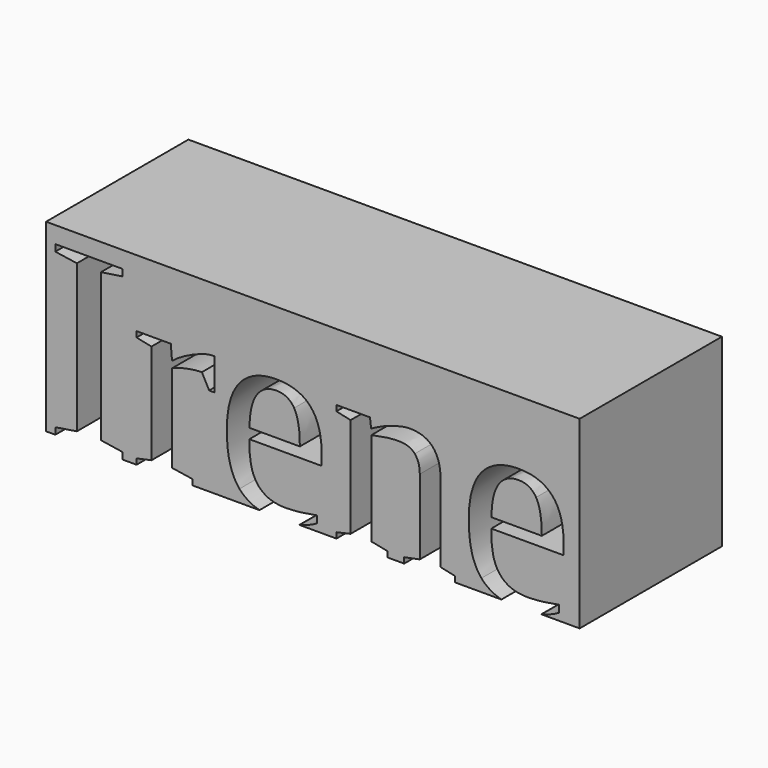
from build123d import *

# Parameters (mm, degrees)
F1_DEPTH = 25.4


with BuildPart() as f1:
    # F0 (on Front) → F1 (new body)
    with BuildSketch(Plane.XZ):
        with BuildLine():
            Line((37.3974812319, 27.1067991487), (-38.8025187681, 27.1067991487))
            Line((-38.8025187681, 27.1067991487), (-38.8025187681, 0.7496755936))
            Line((-38.8025187681, 0.7496755936), (-37.4812306732, 0.7496755936))
            Line((-37.4812306732, 0.7496755936), (-37.4812306732, 1.6991726661))
            Line((-37.4812306732, 1.6991726661), (-34.4039449803, 2.1796410643))
            Line((-34.4039449803, 2.1796410643), (-34.4039449803, 23.3088108586))
            Line((-34.4039449803, 23.3088108586), (-37.4812306732, 23.7721196711))
            Line((-37.4812306732, 23.7721196711), (-37.4812306732, 24.7216167436))
            Line((-37.4812306732, 24.7216167436), (-27.9004620198, 24.7216167436))
            Line((-27.9004620198, 24.7216167436), (-27.9004620198, 23.7721196711))
            Line((-27.9004620198, 23.7721196711), (-30.9720278508, 23.3088108586))
            Line((-30.9720278508, 23.3088108586), (-30.9720278508, 2.1796410643))
            Line((-30.9720278508, 2.1796410643), (-27.9004620198, 1.6991726661))
            Line((-27.9004620198, 1.6991726661), (-27.9004620198, 0.7496755936))
            Line((-27.9004620198, 0.7496755936), (-25.8813507753, 0.7496755936))
            Line((-25.8813507753, 0.7496755936), (-25.8813507753, 1.5561761191))
            Line((-25.8813507753, 1.5561761191), (-23.7535621549, 2.0023253459))
            Line((-23.7535621549, 2.0023253459), (-23.7535621549, 16.3019800524))
            Line((-23.7535621549, 16.3019800524), (-25.8813507753, 16.7481292793))
            Line((-25.8813507753, 16.7481292793), (-25.8813507753, 17.5546298047))
            Line((-25.8813507753, 17.5546298047), (-20.9851490038, 17.5546298047))
            Line((-20.9851490038, 17.5546298047), (-20.8192730092, 15.4611603557))
            add(Edge.make_bspline(
                [(-20.8192730092, 15.4611603557), (-19.7496588371, 16.3534588094), (-17.9164431038, 17.1771189205)],
                knots=[0, 0, 0, 1, 1, 1], degree=2))
            add(Edge.make_bspline(
                [(-17.9164431038, 17.1771189205), (-16.0832273704, 18.0007790316), (-15.0136131983, 18.0007790316)],
                knots=[0, 0, 0, 1, 1, 1], degree=2))
            Line((-15.0136131983, 18.0007790316), (-14.7447796899, 18.0007790316))
            Line((-14.7447796899, 18.0007790316), (-14.7447796899, 13.4592086968))
            Line((-14.7447796899, 13.4592086968), (-15.5112411821, 13.4592086968))
            Line((-15.5112411821, 13.4592086968), (-16.5522560448, 15.4268411844))
            add(Edge.make_bspline(
                [(-16.5522560448, 15.4268411844), (-17.4445544984, 15.4268411844), (-18.6686049413, 15.1837470544)],
                knots=[0, 0, 0, 1, 1, 1], degree=2))
            add(Edge.make_bspline(
                [(-18.6686049413, 15.1837470544), (-19.8926553842, 14.9406529244), (-20.7849538379, 14.5517023164)],
                knots=[0, 0, 0, 1, 1, 1], degree=2))
            Line((-20.7849538379, 14.5517023164), (-20.7849538379, 2.0023253459))
            Line((-20.7849538379, 2.0023253459), (-17.9078633109, 1.5561761191))
            Line((-17.9078633109, 1.5561761191), (-17.9078633109, 0.7496755936))
            Line((-17.9078633109, 0.7496755936), (-8.3285276719, 0.7496755936))
            add(Edge.make_bspline(
                [(-8.3285276719, 0.7496755936), (-10.11731664, 1.2614297437), (-11.181305737, 2.4999533297)],
                knots=[0.4131969353, 0.4131969353, 0.4131969353, 1, 1, 1], degree=2))
            add(Edge.make_bspline(
                [(-11.181305737, 2.4999533297), (-12.9945019538, 4.6105823644), (-12.9945019538, 9.2779896606)],
                knots=[0, 0, 0, 1, 1, 1], degree=2))
            add(Edge.make_bspline(
                [(-12.9945019538, 9.2779896606), (-12.9945019538, 13.6708435864), (-11.1527064276, 15.835811309)],
                knots=[0, 0, 0, 1, 1, 1], degree=2))
            add(Edge.make_bspline(
                [(-11.1527064276, 15.835811309), (-9.3109109014, 18.0007790316), (-5.8961533575, 18.0007790316)],
                knots=[0, 0, 0, 1, 1, 1], degree=2))
            add(Edge.make_bspline(
                [(-5.8961533575, 18.0007790316), (0.5558508461, 18.0007790316), (0.5558508461, 10.6679160981)],
                knots=[0, 0, 0, 1, 1, 1], degree=2))
            Line((0.5558508461, 10.6679160981), (0.5558508461, 9.2036314561))
            Line((0.5558508461, 9.2036314561), (-9.7742197139, 9.2036314561))
            Line((-9.7742197139, 9.2036314561), (-9.7742197139, 8.8833191907))
            add(Edge.make_bspline(
                [(-9.7742197139, 8.8833191907), (-9.7742197139, 6.4180587193), (-9.230832835, 5.0510117294)],
                knots=[0, 0, 0, 1, 1, 1], degree=2))
            add(Edge.make_bspline(
                [(-9.230832835, 5.0510117294), (-8.6874459562, 3.6839647394), (-7.5520533725, 2.9689820041)],
                knots=[0, 0, 0, 1, 1, 1], degree=2))
            add(Edge.make_bspline(
                [(-7.5520533725, 2.9689820041), (-6.4166607888, 2.2539992688), (-4.5748652626, 2.2539992688)],
                knots=[0, 0, 0, 1, 1, 1], degree=2))
            add(Edge.make_bspline(
                [(-4.5748652626, 2.2539992688), (-3.6082086044, 2.2539992688), (-2.2869205095, 2.4141554015)],
                knots=[0, 0, 0, 1, 1, 1], degree=2))
            add(Edge.make_bspline(
                [(-2.2869205095, 2.4141554015), (-0.9656324147, 2.5743115342), (-0.1076531323, 2.7687868382)],
                knots=[0, 0, 0, 1, 1, 1], degree=2))
            Line((-0.1076531323, 2.7687868382), (-0.1076531323, 1.7678110087))
            add(Edge.make_bspline(
                [(-0.1076531323, 1.7678110087), (-0.9656324147, 1.2129844061), (-2.4384968494, 0.8011543506)],
                knots=[0, 0, 0, 1, 1, 1], degree=2))
            add(Edge.make_bspline(
                [(-2.4384968494, 0.8011543506), (-2.5336227612, 0.7745560374), (-2.6290230549, 0.7496755936)],
                knots=[0, 0, 0, 0.0645856533, 0.0645856533, 0.0645856533], degree=2))
            Line((-2.6290230549, 0.7496755936), (2.6664798808, 0.7496755936))
            Line((2.6664798808, 0.7496755936), (2.6664798808, 1.5561761191))
            Line((2.6664798808, 1.5561761191), (4.6855911253, 2.0023253459))
            Line((4.6855911253, 2.0023253459), (4.6855911253, 16.3019800524))
            Line((4.6855911253, 16.3019800524), (2.6664798808, 16.7481292793))
            Line((2.6664798808, 16.7481292793), (2.6664798808, 17.5546298047))
            Line((2.6664798808, 17.5546298047), (7.4540042765, 17.5546298047))
            Line((7.4540042765, 17.5546298047), (7.6198802711, 16.1933026767))
            add(Edge.make_bspline(
                [(7.6198802711, 16.1933026767), (8.9926471229, 16.9826436165), (10.548449555, 17.491711324)],
                knots=[0, 0, 0, 1, 1, 1], degree=2))
            add(Edge.make_bspline(
                [(10.548449555, 17.491711324), (12.1042519871, 18.0007790316), (13.1395469878, 18.0007790316)],
                knots=[0, 0, 0, 1, 1, 1], degree=2))
            add(Edge.make_bspline(
                [(13.1395469878, 18.0007790316), (15.3188143651, 18.0007790316), (16.4284675703, 16.7309696936)],
                knots=[0, 0, 0, 1, 1, 1], degree=2))
            add(Edge.make_bspline(
                [(16.4284675703, 16.7309696936), (17.5381207755, 15.4611603557), (17.5381207755, 13.0473786412)],
                knots=[0, 0, 0, 1, 1, 1], degree=2))
            Line((17.5381207755, 13.0473786412), (17.5381207755, 2.0023253459))
            Line((17.5381207755, 2.0023253459), (19.5743916057, 1.5561761191))
            Line((19.5743916057, 1.5561761191), (19.5743916057, 0.7496755936))
            Line((19.5743916057, 0.7496755936), (26.2251579609, 0.7496755936))
            add(Edge.make_bspline(
                [(26.2251579609, 0.7496755936), (24.4363689928, 1.2614297437), (23.3723798958, 2.4999533297)],
                knots=[0.4131969353, 0.4131969353, 0.4131969353, 1, 1, 1], degree=2))
            add(Edge.make_bspline(
                [(23.3723798958, 2.4999533297), (21.559183679, 4.6105823644), (21.559183679, 9.2779896606)],
                knots=[0, 0, 0, 1, 1, 1], degree=2))
            add(Edge.make_bspline(
                [(21.559183679, 9.2779896606), (21.559183679, 13.6708435864), (23.4009792052, 15.835811309)],
                knots=[0, 0, 0, 1, 1, 1], degree=2))
            add(Edge.make_bspline(
                [(23.4009792052, 15.835811309), (25.2427747314, 18.0007790316), (28.6575322753, 18.0007790316)],
                knots=[0, 0, 0, 1, 1, 1], degree=2))
            add(Edge.make_bspline(
                [(28.6575322753, 18.0007790316), (35.1095364789, 18.0007790316), (35.1095364789, 10.6679160981)],
                knots=[0, 0, 0, 1, 1, 1], degree=2))
            Line((35.1095364789, 10.6679160981), (35.1095364789, 9.2036314561))
            Line((35.1095364789, 9.2036314561), (24.7794659189, 9.2036314561))
            Line((24.7794659189, 9.2036314561), (24.7794659189, 8.8833191907))
            add(Edge.make_bspline(
                [(24.7794659189, 8.8833191907), (24.7794659189, 6.4180587193), (25.3228527978, 5.0510117294)],
                knots=[0, 0, 0, 1, 1, 1], degree=2))
            add(Edge.make_bspline(
                [(25.3228527978, 5.0510117294), (25.8662396766, 3.6839647394), (27.0016322603, 2.9689820041)],
                knots=[0, 0, 0, 1, 1, 1], degree=2))
            add(Edge.make_bspline(
                [(27.0016322603, 2.9689820041), (28.137024844, 2.2539992688), (29.9788203702, 2.2539992688)],
                knots=[0, 0, 0, 1, 1, 1], degree=2))
            add(Edge.make_bspline(
                [(29.9788203702, 2.2539992688), (30.9454770284, 2.2539992688), (32.2667651232, 2.4141554015)],
                knots=[0, 0, 0, 1, 1, 1], degree=2))
            add(Edge.make_bspline(
                [(32.2667651232, 2.4141554015), (33.5880532181, 2.5743115342), (34.4460325005, 2.7687868382)],
                knots=[0, 0, 0, 1, 1, 1], degree=2))
            Line((34.4460325005, 2.7687868382), (34.4460325005, 1.7678110087))
            add(Edge.make_bspline(
                [(34.4460325005, 1.7678110087), (33.5880532181, 1.2129844061), (32.1151887834, 0.8011543506)],
                knots=[0, 0, 0, 1, 1, 1], degree=2))
            add(Edge.make_bspline(
                [(32.1151887834, 0.8011543506), (32.0200628716, 0.7745560374), (31.9246625779, 0.7496755936)],
                knots=[0, 0, 0, 0.0645856533, 0.0645856533, 0.0645856533], degree=2))
            Line((31.9246625779, 0.7496755936), (37.3974812319, 0.7496755936))
            Line((37.3974812319, 0.7496755936), (37.3974812319, 27.1067991487))
        make_face()
    extrude(amount=F1_DEPTH)


with BuildPart() as f1b:
    # F0 (on Front) → F1, piece 2 (new body)
    with BuildSketch(Plane.XZ):
        with BuildLine():
            Line((9.9249846098, 0.7496755936), (12.3387663243, 0.7496755936))
            Line((12.3387663243, 0.7496755936), (12.3387663243, 1.5561761191))
            Line((12.3387663243, 1.5561761191), (14.5695124585, 2.0023253459))
            Line((14.5695124585, 2.0023253459), (14.5695124585, 12.7270663758))
            add(Edge.make_bspline(
                [(14.5695124585, 12.7270663758), (14.5695124585, 14.2085106034), (13.8459499303, 15.057910093)],
                knots=[0, 0, 0, 1, 1, 1], degree=2))
            add(Edge.make_bspline(
                [(13.8459499303, 15.057910093), (13.1223874022, 15.9073095825), (11.6009041414, 15.9073095825)],
                knots=[0, 0, 0, 1, 1, 1], degree=2))
            add(Edge.make_bspline(
                [(11.6009041414, 15.9073095825), (9.9936229524, 15.9073095825), (7.6541994424, 15.3868021512)],
                knots=[0, 0, 0, 1, 1, 1], degree=2))
            Line((7.6541994424, 15.3868021512), (7.6541994424, 2.0023253459))
            Line((7.6541994424, 2.0023253459), (9.9249846098, 1.5561761191))
            Line((9.9249846098, 1.5561761191), (9.9249846098, 0.7496755936))
        make_face()
    extrude(amount=F1_DEPTH)


with BuildPart() as f1c:
    # F0 (on Front) → F1, piece 3 (new body)
    with BuildSketch(Plane.XZ):
        with BuildLine():
            add(Edge.make_bspline(
                [(31.1771314346, 15.203766571), (30.3563312545, 16.5708135609), (28.6575322753, 16.5708135609)],
                knots=[0, 0, 0, 1, 1, 1], degree=2))
            add(Edge.make_bspline(
                [(28.6575322753, 16.5708135609), (26.7985771635, 16.5708135609), (25.8061811268, 15.0693498167)],
                knots=[0, 0, 0, 1, 1, 1], degree=2))
            add(Edge.make_bspline(
                [(25.8061811268, 15.0693498167), (24.8137850902, 13.5678860725), (24.8137850902, 10.6335969268)],
                knots=[0, 0, 0, 1, 1, 1], degree=2))
            Line((24.8137850902, 10.6335969268), (31.9979316148, 10.6335969268))
            add(Edge.make_bspline(
                [(31.9979316148, 10.6335969268), (31.9979316148, 13.836719581), (31.1771314346, 15.203766571)],
                knots=[0, 0, 0, 1, 1, 1], degree=2))
        make_face()
    extrude(amount=F1_DEPTH)


with BuildPart() as f1d:
    # F0 (on Front) → F1, piece 4 (new body)
    with BuildSketch(Plane.XZ):
        with BuildLine():
            add(Edge.make_bspline(
                [(-3.3765541982, 15.203766571), (-4.1973543783, 16.5708135609), (-5.8961533575, 16.5708135609)],
                knots=[0, 0, 0, 1, 1, 1], degree=2))
            add(Edge.make_bspline(
                [(-5.8961533575, 16.5708135609), (-7.7551084693, 16.5708135609), (-8.7475045059, 15.0693498167)],
                knots=[0, 0, 0, 1, 1, 1], degree=2))
            add(Edge.make_bspline(
                [(-8.7475045059, 15.0693498167), (-9.7399005426, 13.5678860725), (-9.7399005426, 10.6335969268)],
                knots=[0, 0, 0, 1, 1, 1], degree=2))
            Line((-9.7399005426, 10.6335969268), (-2.555754018, 10.6335969268))
            add(Edge.make_bspline(
                [(-2.555754018, 10.6335969268), (-2.555754018, 13.836719581), (-3.3765541982, 15.203766571)],
                knots=[0, 0, 0, 1, 1, 1], degree=2))
        make_face()
    extrude(amount=F1_DEPTH)


solid = Compound([f1.part, f1b.part, f1c.part, f1d.part])
